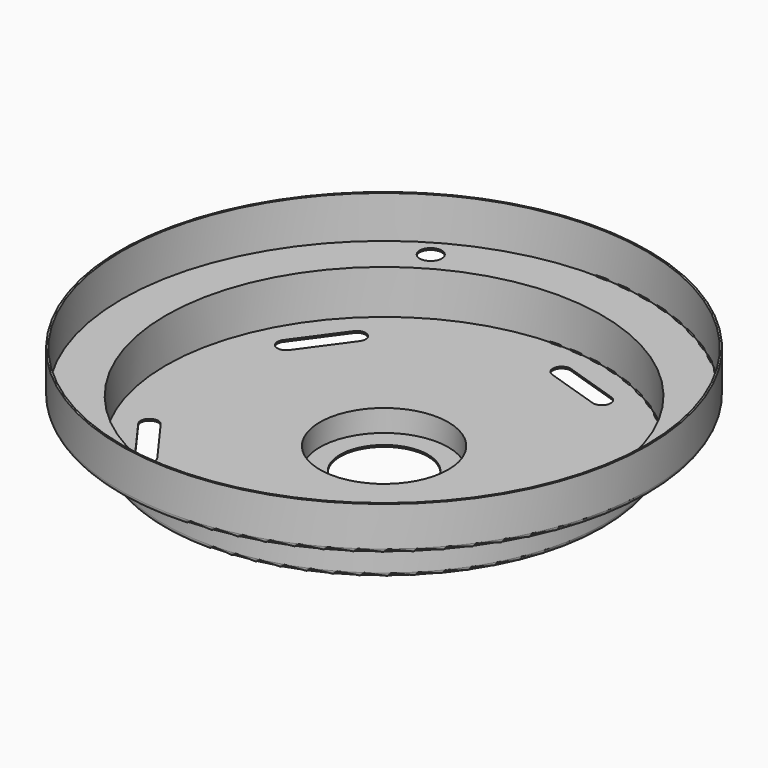
from build123d import *

# Parameters (mm, degrees)
F2_R            = 3.175
F3_DEPTH        = 19.559
F3_COPIES_COUNT = 3
F5_DEPTH        = 6.859
F5_COPIES_COUNT = 5
F6_R            = 1.27


# Not quite as in the source:
# - a pattern or mirror of a feature is missing from the dataset's text; its kind, count and spacing are read off the source's solid


with BuildPart() as f1:
    # F0 (on Front) → F1 (revolve)
    with BuildSketch(Plane.XZ):
        Polygon((0, 0.508), (0, 0), (6.35, 0), (6.35, 6.35), (50.8, 6.35), (50.8, 19.05), (63.5, 19.05), (63.5, 31.75), (62.992, 31.75), (62.992, 19.558), (50.292, 19.558), (50.292, 6.858), (5.842, 6.858), (5.842, 0.508), align=None)
    revolve(axis=Axis((-12.7, 0, 6.35), (0, 0, 1)))

    # F2 (on face) → F3 (cut, through all)
    with BuildSketch(Plane.XY.offset(19.558)):
        with Locations((57.15, 0)):
            Circle(F2_R)
    f3 = extrude(amount=-F3_DEPTH, mode=Mode.SUBTRACT)

    # F3_copies: F3 ×3 about axis
    f3_copies_axis = Axis((-12.7, 0, 0), (0, 0, 1))
    for i in range(1, F3_COPIES_COUNT):
        add(f3.rotate(f3_copies_axis, i * 360 / F3_COPIES_COUNT), mode=Mode.SUBTRACT)

    # F4 (on face) → F5 (cut, through all)
    with BuildSketch(Plane.XY.offset(6.858)):
        with BuildLine():
            ThreePointArc((43.18, 8.255), (40.64, 10.795), (38.1, 8.255))
            Line((38.1, 8.255), (43.18, 8.255))
        make_face()
        Polygon((38.1, 8.255), (38.1, 0), (38.1, -8.255), (43.18, -8.255), (43.18, 8.255), align=None)
        with BuildLine():
            Line((43.18, -8.255), (38.1, -8.255))
            ThreePointArc((38.1, -8.255), (40.64, -10.795), (43.18, -8.255))
        make_face()
    f5 = extrude(amount=-F5_DEPTH, mode=Mode.SUBTRACT)

    # F5_copies: F5 ×5 about axis
    f5_copies_axis = Axis((-12.7, 0, 0), (0, 0, 1))
    for i in range(1, F5_COPIES_COUNT):
        add(f5.rotate(f5_copies_axis, i * 360 / F5_COPIES_COUNT), mode=Mode.SUBTRACT)

    # F6
    f6_edges = [f1.edges().sort_by_distance(p)[0] for p in [
        (-88.9, 0, 19.05),
        (-76.2, 0, 19.05),
        (-76.2, 0, 6.35),
        (-31.75, 0, 6.35),
        (-31.75, 0, 0),
    ]]
    fillet(f6_edges, radius=F6_R)


solid = f1.part
